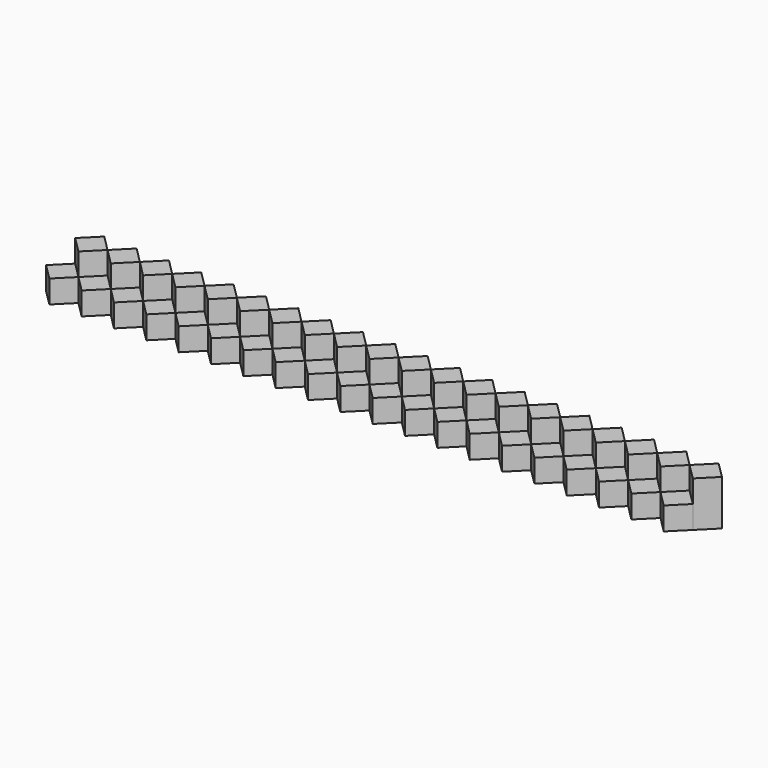
from build123d import *

# Parameters (mm, degrees)
F1_DEPTH = 7.07107
F2_DEPTH = 14.034


with BuildPart() as f1:
    # F0 (on Top) → F1 (new body)
    with BuildSketch(Plane.XY):
        Polygon((5, 0), (0, 5), (-5, 0), (0, -5), align=None)
    extrude(amount=F1_DEPTH)

    # F0 (on Top) → F2, piece 4 (join)
    with BuildSketch(Plane.XY):
        Polygon((5, 10), (0, 5), (5, 0), (10, 5), align=None)
    extrude(amount=F2_DEPTH)


with BuildPart() as f1b:
    # F0 (on Top) → F1, piece 2 (new body)
    with BuildSketch(Plane.XY):
        Polygon((10, 5), (5, 0), (10, -5), (15, 0), align=None)
    extrude(amount=F1_DEPTH)

    # F0 (on Top) → F2 (join)
    with BuildSketch(Plane.XY):
        Polygon((15, 10), (10, 5), (15, 0), (20, 5), align=None)
    extrude(amount=F2_DEPTH)


with BuildPart() as f1c:
    # F0 (on Top) → F1, piece 3 (new body)
    with BuildSketch(Plane.XY):
        Polygon((20, 5), (15, 0), (20, -5), (25, 0), align=None)
    extrude(amount=F1_DEPTH)



with BuildPart() as f1d:
    # F0 (on Top) → F1, piece 4 (new body)
    with BuildSketch(Plane.XY):
        Polygon((30, 5), (25, 0), (30, -5), (35, 0), align=None)
    extrude(amount=F1_DEPTH)


with BuildPart() as f1e:
    # F0 (on Top) → F1, piece 5 (new body)
    with BuildSketch(Plane.XY):
        Polygon((40, 5), (35, 0), (40, -5), (45, 0), align=None)
    extrude(amount=F1_DEPTH)



with BuildPart() as f1f:
    # F0 (on Top) → F1, piece 6 (new body)
    with BuildSketch(Plane.XY):
        Polygon((50, 5), (45, 0), (50, -5), (55, 0), align=None)
    extrude(amount=F1_DEPTH)


with BuildPart() as f1g:
    # F0 (on Top) → F1, piece 7 (new body)
    with BuildSketch(Plane.XY):
        Polygon((60, 5), (55, 0), (60, -5), (65, 0), align=None)
    extrude(amount=F1_DEPTH)



with BuildPart() as f1h:
    # F0 (on Top) → F1, piece 8 (new body)
    with BuildSketch(Plane.XY):
        Polygon((70, 5), (65, 0), (70, -5), (75, 0), align=None)
    extrude(amount=F1_DEPTH)


with BuildPart() as f1i:
    # F0 (on Top) → F1, piece 9 (new body)
    with BuildSketch(Plane.XY):
        Polygon((80, 5), (75, 0), (80, -5), (85, 0), align=None)
    extrude(amount=F1_DEPTH)



with BuildPart() as f1j:
    # F0 (on Top) → F1, piece 10 (new body)
    with BuildSketch(Plane.XY):
        Polygon((90, 5), (85, 0), (90, -5), (95, 0), align=None)
    extrude(amount=F1_DEPTH)


with BuildPart() as f1k:
    # F0 (on Top) → F1, piece 11 (new body)
    with BuildSketch(Plane.XY):
        Polygon((100, 5), (95, 0), (100, -5), (105, 0), align=None)
    extrude(amount=F1_DEPTH)



with BuildPart() as f1l:
    # F0 (on Top) → F1, piece 12 (new body)
    with BuildSketch(Plane.XY):
        Polygon((110, 5), (105, 0), (110, -5), (115, 0), align=None)
    extrude(amount=F1_DEPTH)


with BuildPart() as f1m:
    # F0 (on Top) → F1, piece 13 (new body)
    with BuildSketch(Plane.XY):
        Polygon((120, 5), (115, 0), (120, -5), (125, 0), align=None)
    extrude(amount=F1_DEPTH)



with BuildPart() as f1n:
    # F0 (on Top) → F1, piece 14 (new body)
    with BuildSketch(Plane.XY):
        Polygon((130, 5), (125, 0), (130, -5), (135, 0), align=None)
    extrude(amount=F1_DEPTH)


with BuildPart() as f1o:
    # F0 (on Top) → F1, piece 15 (new body)
    with BuildSketch(Plane.XY):
        Polygon((140, 5), (135, 0), (140, -5), (145, 0), align=None)
    extrude(amount=F1_DEPTH)



with BuildPart() as f1p:
    # F0 (on Top) → F1, piece 16 (new body)
    with BuildSketch(Plane.XY):
        Polygon((150, 5), (145, 0), (150, -5), (155, 0), align=None)
    extrude(amount=F1_DEPTH)


with BuildPart() as f1q:
    # F0 (on Top) → F1, piece 17 (new body)
    with BuildSketch(Plane.XY):
        Polygon((160, 5), (155, 0), (160, -5), (165, 0), align=None)
    extrude(amount=F1_DEPTH)



with BuildPart() as f1r:
    # F0 (on Top) → F1, piece 18 (new body)
    with BuildSketch(Plane.XY):
        Polygon((170, 5), (165, 0), (170, -5), (175, 0), align=None)
    extrude(amount=F1_DEPTH)


with BuildPart() as f1s:
    # F0 (on Top) → F1, piece 19 (new body)
    with BuildSketch(Plane.XY):
        Polygon((180, 5), (175, 0), (180, -5), (185, 0), align=None)
    extrude(amount=F1_DEPTH)



with BuildPart() as f1t:
    # F0 (on Top) → F1, piece 20 (new body)
    with BuildSketch(Plane.XY):
        Polygon((190, 5), (185, 0), (190, -5), (195, 0), align=None)
    extrude(amount=F1_DEPTH)


with BuildPart() as f1c_1:
    add(f1c.part)

    add(f1d.part)  # F2#2 merges F1d
    # F0 (on Top) → F2, piece 2 (join)
    with BuildSketch(Plane.XY):
        Polygon((25, 10), (20, 5), (25, 0), (30, 5), align=None)
    extrude(amount=F2_DEPTH)


with BuildPart() as f2:
    # F0 (on Top) → F2, piece 3 (new body)
    with BuildSketch(Plane.XY):
        Polygon((35, 10), (30, 5), (35, 0), (40, 5), align=None)
    extrude(amount=F2_DEPTH)


with BuildPart() as f1e_1:
    add(f1e.part)

    add(f1f.part)  # F2#5 merges F1f
    # F0 (on Top) → F2, piece 5 (join)
    with BuildSketch(Plane.XY):
        Polygon((45, 10), (40, 5), (45, 0), (50, 5), align=None)
    extrude(amount=F2_DEPTH)


with BuildPart() as f2b:
    # F0 (on Top) → F2, piece 6 (new body)
    with BuildSketch(Plane.XY):
        Polygon((95, 10), (90, 5), (95, 0), (100, 5), align=None)
    extrude(amount=F2_DEPTH)


with BuildPart() as f1k_1:
    add(f1k.part)

    add(f1l.part)  # F2#7 merges F1l
    # F0 (on Top) → F2, piece 7 (join)
    with BuildSketch(Plane.XY):
        Polygon((105, 10), (100, 5), (105, 0), (110, 5), align=None)
    extrude(amount=F2_DEPTH)


with BuildPart() as f2c:
    # F0 (on Top) → F2, piece 8 (new body)
    with BuildSketch(Plane.XY):
        Polygon((115, 10), (110, 5), (115, 0), (120, 5), align=None)
    extrude(amount=F2_DEPTH)


with BuildPart() as f1m_1:
    add(f1m.part)

    add(f1n.part)  # F2#9 merges F1n
    # F0 (on Top) → F2, piece 9 (join)
    with BuildSketch(Plane.XY):
        Polygon((125, 10), (120, 5), (125, 0), (130, 5), align=None)
    extrude(amount=F2_DEPTH)


with BuildPart() as f2d:
    # F0 (on Top) → F2, piece 10 (new body)
    with BuildSketch(Plane.XY):
        Polygon((135, 10), (130, 5), (135, 0), (140, 5), align=None)
    extrude(amount=F2_DEPTH)


with BuildPart() as f1o_1:
    add(f1o.part)

    add(f1p.part)  # F2#11 merges F1p
    # F0 (on Top) → F2, piece 11 (join)
    with BuildSketch(Plane.XY):
        Polygon((145, 10), (140, 5), (145, 0), (150, 5), align=None)
    extrude(amount=F2_DEPTH)


with BuildPart() as f2e:
    # F0 (on Top) → F2, piece 12 (new body)
    with BuildSketch(Plane.XY):
        Polygon((155, 10), (150, 5), (155, 0), (160, 5), align=None)
    extrude(amount=F2_DEPTH)


with BuildPart() as f1q_1:
    add(f1q.part)

    add(f1r.part)  # F2#13 merges F1r
    # F0 (on Top) → F2, piece 13 (join)
    with BuildSketch(Plane.XY):
        Polygon((165, 10), (160, 5), (165, 0), (170, 5), align=None)
    extrude(amount=F2_DEPTH)


with BuildPart() as f2f:
    # F0 (on Top) → F2, piece 14 (new body)
    with BuildSketch(Plane.XY):
        Polygon((175, 10), (170, 5), (175, 0), (180, 5), align=None)
    extrude(amount=F2_DEPTH)


with BuildPart() as f1s_1:
    add(f1s.part)

    add(f1t.part)  # F2#15 merges F1t
    # F0 (on Top) → F2, piece 15 (join)
    with BuildSketch(Plane.XY):
        Polygon((185, 10), (180, 5), (185, 0), (190, 5), align=None)
    extrude(amount=F2_DEPTH)


with BuildPart() as f2g:
    # F0 (on Top) → F2, piece 16 (new body)
    with BuildSketch(Plane.XY):
        Polygon((195, 10), (190, 5), (195, 0), (200, 5), align=None)
    extrude(amount=F2_DEPTH)


with BuildPart() as f1i_1:
    add(f1i.part)

    add(f1j.part)  # F2#17 merges F1j
    # F0 (on Top) → F2, piece 17 (join)
    with BuildSketch(Plane.XY):
        Polygon((85, 10), (80, 5), (85, 0), (90, 5), align=None)
    extrude(amount=F2_DEPTH)


with BuildPart() as f2h:
    # F0 (on Top) → F2, piece 18 (new body)
    with BuildSketch(Plane.XY):
        Polygon((75, 10), (70, 5), (75, 0), (80, 5), align=None)
    extrude(amount=F2_DEPTH)


with BuildPart() as f2i:
    # F0 (on Top) → F2, piece 19 (new body)
    with BuildSketch(Plane.XY):
        Polygon((55, 10), (50, 5), (55, 0), (60, 5), align=None)
    extrude(amount=F2_DEPTH)


with BuildPart() as f1g_1:
    add(f1g.part)

    add(f1h.part)  # F2#20 merges F1h
    # F0 (on Top) → F2, piece 20 (join)
    with BuildSketch(Plane.XY):
        Polygon((65, 10), (60, 5), (65, 0), (70, 5), align=None)
    extrude(amount=F2_DEPTH)


solid = Compound([f1.part, f1b.part, f1c_1.part, f2.part, f1e_1.part, f2b.part, f1k_1.part, f2c.part, f1m_1.part, f2d.part, f1o_1.part, f2e.part, f1q_1.part, f2f.part, f1s_1.part, f2g.part, f1i_1.part, f2h.part, f2i.part, f1g_1.part])
